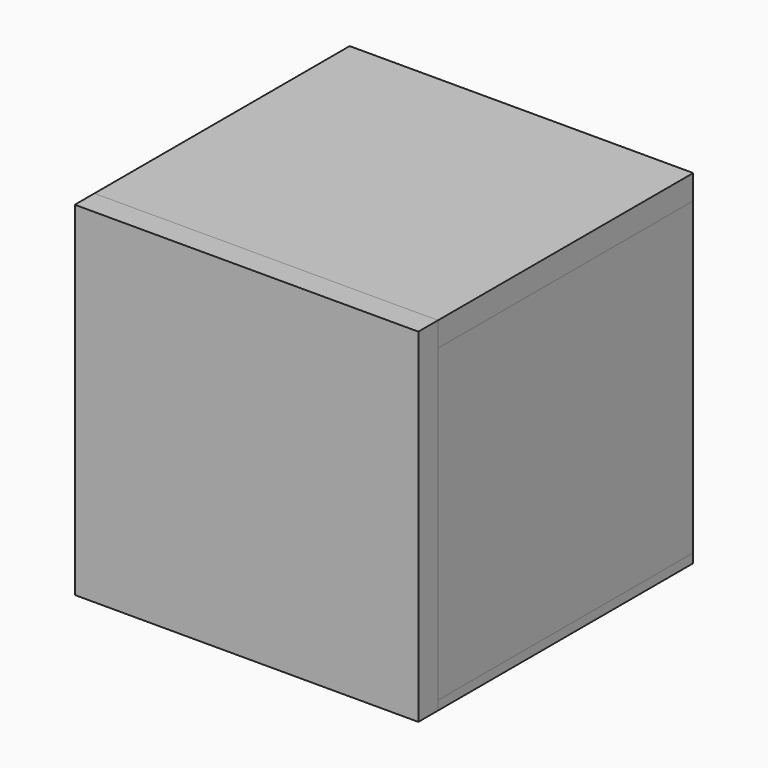
from build123d import *

# Parameters (mm, degrees)
F0_W      = 168
F0_H      = 168
F1_DEPTH  = 12
F2_W      = 156
F2_H      = 151.5
F3_DEPTH  = 12
F5_W      = 168
F5_H      = 156
F6_DEPTH  = 12
F7_W      = 168
F7_H      = 156
F8_DEPTH  = 4.5
F9_W      = 130
F9_H      = 130
F10_DEPTH = 4.5
F11_W     = 3
F11_H     = 3
F12_DEPTH = 142
F14_W     = 150
F14_H     = 150
F15_DEPTH = 3


# Not quite as in the source:
# - a feature names something its author has since deleted; it is built from what else it names


with BuildPart() as f1:
    # F0 (on Front) → F1 (new body)
    with BuildSketch(Plane.XZ):
        with Locations((0, 0.5)):
            Rectangle(F0_W, F0_H)
    extrude(amount=F1_DEPTH)


with BuildPart() as f3:
    # F2 (on face) → F3 (new body)
    with BuildSketch(Plane.YZ.offset(84)):
        with Locations((78, -3.25)):
            Rectangle(F2_W, F2_H)
    extrude(amount=-F3_DEPTH)

    # F11 (on face) → F12 (cut)
    with BuildSketch(Plane(origin=(0, 156, 0), x_dir=(-1, 0, 0), z_dir=(0, 1, 0))):
        with Locations((-73.5, 0.5)):
            Rectangle(F11_W, F11_H)
        with Locations((-73.5, -42.5)):
            Rectangle(F11_W, F11_H)
    extrude(amount=-F12_DEPTH, mode=Mode.SUBTRACT)


with BuildPart() as f4_1:
    # F4: instance of F1
    add(f1.part.mirror(Plane.YZ))


with BuildPart() as f6:
    # F5 (on face) → F6 (new body)
    with BuildSketch(Plane.XY.offset(84.5)):
        with Locations((0, 78)):
            Rectangle(F5_W, F5_H)
    extrude(amount=-F6_DEPTH)


with BuildPart() as f8:
    # F7 (on face) → F8 (new body)
    with BuildSketch(Plane(origin=(0, 0, -83.5), x_dir=(1, 0, 0), z_dir=(0, 0, -1))):
        with Locations((0, -78)):
            Rectangle(F7_W, F7_H)
    extrude(amount=-F8_DEPTH)


with BuildPart() as f10:
    # F9 (on face) → F10 (new body)
    with BuildSketch(Plane(origin=(0, 156, 0), x_dir=(-1, 0, 0), z_dir=(0, 1, 0))):
        with Locations((-7, 7.5)):
            Rectangle(F9_W, F9_H)
    extrude(amount=-F10_DEPTH)


with BuildPart() as f13_1:
    # F13: instance of F3
    add(f3.part.mirror(Plane.YZ))


with BuildPart() as f15:
    # F14 (on face) → F15 (new body)
    with BuildSketch(Plane.XY.offset(-1)):
        with Locations((0, 75)):
            Rectangle(F14_W, F14_H)
    extrude(amount=F15_DEPTH)


with BuildPart() as f16_1:
    # F16: copy of F15
    add(f15.part.moved(Location((0, 0, -43))))


solid = Compound([f1.part, f3.part, f4_1.part, f6.part, f8.part, f10.part, f13_1.part, f15.part, f16_1.part])
